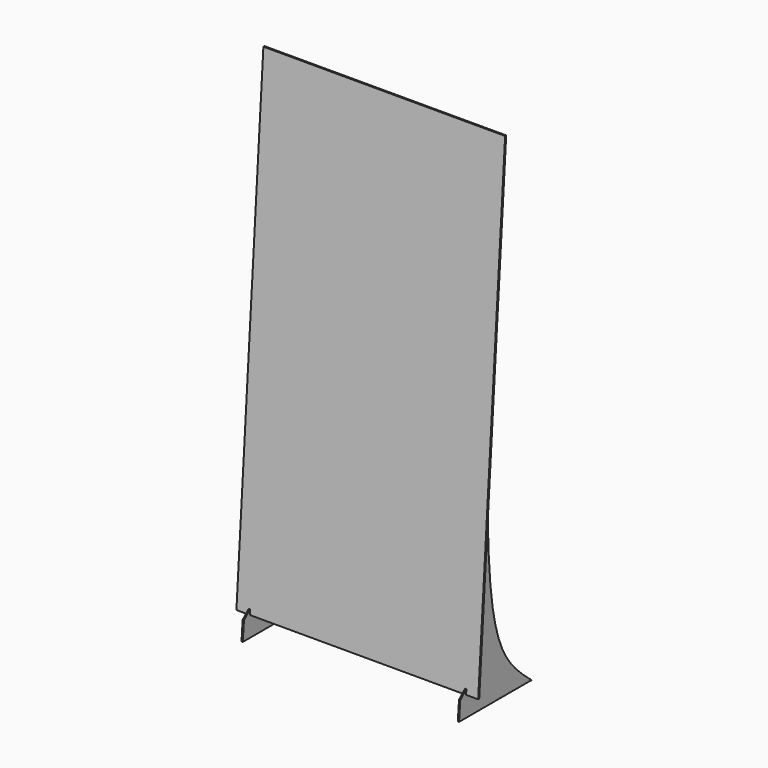
from build123d import *

# Parameters (mm, degrees)
F2_DEPTH = 609.6
F3_START = 542.29
F3_DEPTH = 6.35


# Not quite as in the source:
# - a length typed as a fraction of an inch, garbled in the dataset ("3 / 203.2 mm" for 3/8 in), is restored


with BuildPart() as f2:
    # F0 (on Right) → F2 (new body, symmetric)
    with BuildSketch(Plane.YZ):
        Polygon((-6.5879129879, 0.4606717526), (0, 0), (170.0941855777, 2432.4601801536), (163.4740592827, 2432.4601801536), align=None)
    extrude(amount=F2_DEPTH, both=True)

    # F1 (on Right) → F3 (join)
    with BuildSketch(Plane.YZ.offset(F3_START)):
        with BuildLine():
            Line((-43.1832319469, -7.9277986727), (-50.8, -101.6))
            Line((-50.8, -101.6), (406.4, -101.6))
            add(Edge.make_bspline(
                [(128.1419030371, 1060.091129987), (120.5565482378, 184.9341541529), (188.3697360754, 77.5789916515), (406.4, -101.6)],
                knots=[0, 0, 0, 0, 1194.5517360148, 1194.5517360148, 1194.5517360148, 1194.5517360148], degree=3))
            Line((128.1419030371, 1060.091129987), (78.1502050281, 1117.6))
            Line((78.1502050281, 1117.6), (0, 0))
            Line((0, 0), (-6.5879129879, 0.4606717526))
            Line((-6.5879129879, 0.4606717526), (-4.8439852716, 25.4))
            Line((-4.8439852716, 25.4), (-43.1832319469, -7.9277986727))
        make_face()
    extrude(amount=F3_DEPTH)

    # F4: F2 across plane


with BuildPart() as f2_1:
    add(f2.part)
    add(f2.part.mirror(Plane.YZ))


solid = f2_1.part
